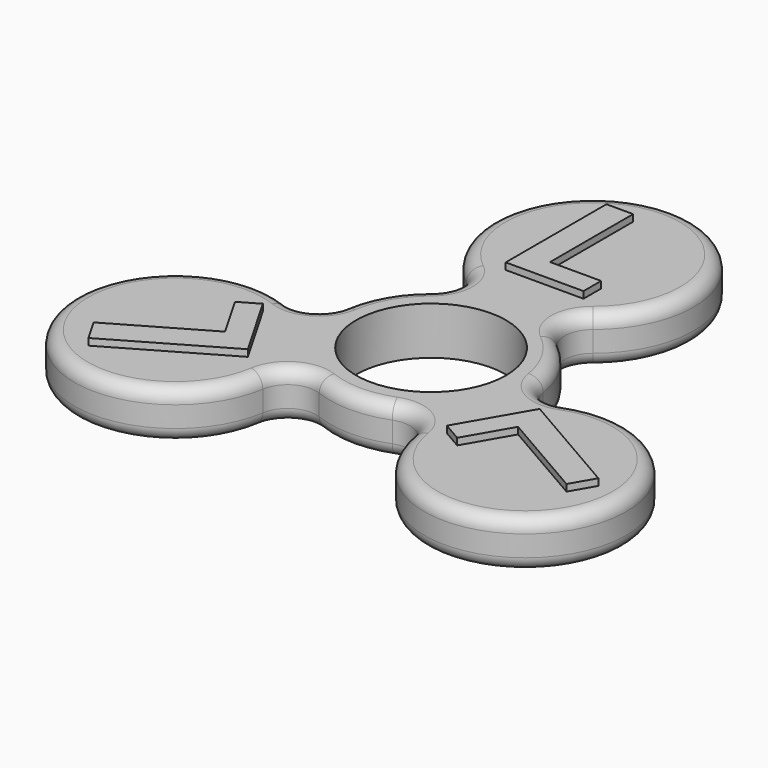
from build123d import *

# Parameters (mm, degrees)
F0_R         = 15
F0_R_2       = 11.125
F1_DEPTH     = 7.1
F3_DEPTH     = 7.1
F4_TEXT_SIZE = 26.1942674923
F5_DEPTH     = 1
F7_COUNT     = 3
F8_R         = 2
F9_R         = 2


# Not quite as in the source:
# - Text() gives the source's letters only with a copy of the font that has no kerning and outlines rounded to 1/6400 em; it was checked with that copy


with BuildPart() as f1:
    # F0 (on Top) → F1 (new body)
    with BuildSketch(Plane.XY):
        Circle(F0_R)
        Circle(F0_R_2, mode=Mode.SUBTRACT)
    extrude(amount=F1_DEPTH)

    # F2 (on Top) → F3 (join)
    with BuildSketch(Plane.XY):
        with BuildLine():
            ThreePointArc((-9.3999616935, 18.3106578388), (-7.8139177176, 15), (-9.3999616935, 11.6893421612))
            ThreePointArc((-9.3999616935, 11.6893421612), (0, 15), (9.3999616935, 11.6893421612))
            ThreePointArc((9.3999616935, 11.6893421612), (7.8139177176, 15), (9.3999616935, 18.3106578388))
            ThreePointArc((9.3999616935, 18.3106578388), (0, 45), (-9.3999616935, 18.3106578388))
        make_face()
        with BuildLine():
            ThreePointArc((-11.1575140017, -17.2959345406), (-9.083422198, -14.2670512465), (-5.4232864184, -13.9852767017))
            ThreePointArc((-5.4232864184, -13.9852767017), (-12.9903810568, -7.5), (-14.8232481118, 2.2959345406))
            ThreePointArc((-14.8232481118, 2.2959345406), (-16.8973399155, -0.7329487535), (-20.5574756952, -1.0147232983))
            ThreePointArc((-20.5574756952, -1.0147232983), (-38.9711431703, -22.5), (-11.1575140017, -17.2959345406))
        make_face()
        with BuildLine():
            ThreePointArc((20.5574756952, -1.0147232983), (16.8973399155, -0.7329487535), (14.8232481118, 2.2959345406))
            ThreePointArc((14.8232481118, 2.2959345406), (12.9903810568, -7.5), (5.4232864184, -13.9852767017))
            ThreePointArc((5.4232864184, -13.9852767017), (9.083422198, -14.2670512465), (11.1575140017, -17.2959345406))
            ThreePointArc((11.1575140017, -17.2959345406), (38.9711431703, -22.5), (20.5574756952, -1.0147232983))
        make_face()
    extrude(amount=F3_DEPTH)

    # F8
    f8_edges = [f1.edges().sort_by_distance(p)[0] for p in [
        (38.971143, -22.5, 7.1),
    ]]
    fillet(f8_edges, radius=F8_R)

    # F9
    f9_edges = [f1.edges().sort_by_distance(p)[0] for p in [
        (-38.971143, -22.5, 0),
    ]]
    fillet(f9_edges, radius=F9_R)


with BuildPart() as f5:
    # F4 (on face) → F5 (new body)
    with BuildSketch(Plane.XY.offset(7.1)):
        with Locations((-7.8009802876, 20.6656064838)):
            Text('L', F4_TEXT_SIZE, font='Open Sans', font_style=FontStyle.BOLD, text_align=(TextAlign.LEFT, TextAlign.BOTTOM))
    extrude(amount=F5_DEPTH)


with BuildPart() as f7_1:
    # F7: instance of F5
    add(f5.part.rotate(Axis((0, 0, 27.481187135), (0, 0, 1)), 1 * 360 / F7_COUNT))


with BuildPart() as f7_2:
    # F7: instance of F5
    add(f5.part.rotate(Axis((0, 0, 27.481187135), (0, 0, 1)), 2 * 360 / F7_COUNT))


solid = Compound([f1.part, f5.part, f7_1.part, f7_2.part])
